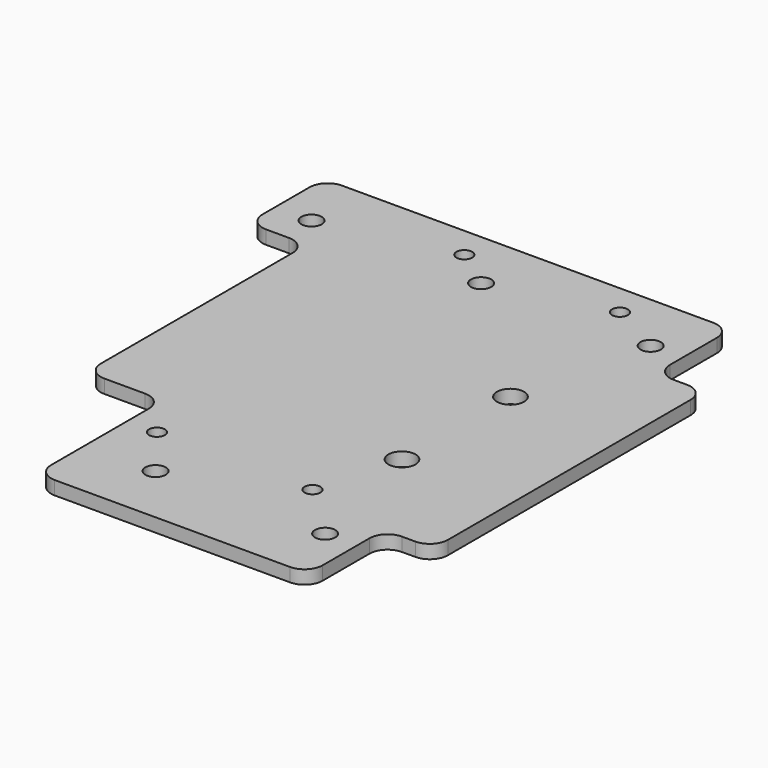
from build123d import *

# Parameters (mm, degrees)
F1_R     = 2.25
F1_R_2   = 1.75
F1_R_3   = 3
F2_DEPTH = 3
F3_W     = 17
F3_H     = 35
F4_DEPTH = 3.001
F5_R     = 4


with BuildPart() as f2:
    # F1 (on Top) → F2 (new body)
    with BuildSketch(Plane.XY):
        Polygon((44.55, 58.5), (-32.5, 58.5), (-45.55, 58.5), (-45.55, 37.5), (-32.5, 37.5), (-32.5, 0), (-32.5, -58.5), (44.55, -58.5), (44.55, -37.55), (55.5, -37.55), (55.5, 37.55), (44.55, 37.55), align=None)
        with Locations((0, -45)):
            Circle(F1_R, mode=Mode.SUBTRACT)
        with Locations((-8.9, -33.5)):
            Circle(F1_R_2, mode=Mode.SUBTRACT)
        with Locations((25.5, -33.5)):
            Circle(F1_R_2, mode=Mode.SUBTRACT)
        with Locations((37.5, -45)):
            Circle(F1_R, mode=Mode.SUBTRACT)
        with Locations((30.5, -15)):
            Circle(F1_R_3, mode=Mode.SUBTRACT)
        with Locations((-37.5, 45)):
            Circle(F1_R, mode=Mode.SUBTRACT)
        with Locations((-8.9, 51.5)):
            Circle(F1_R_2, mode=Mode.SUBTRACT)
        with Locations((0, 45)):
            Circle(F1_R, mode=Mode.SUBTRACT)
        with Locations((30.5, 15)):
            Circle(F1_R_3, mode=Mode.SUBTRACT)
        with Locations((25.5, 51.5)):
            Circle(F1_R_2, mode=Mode.SUBTRACT)
        with Locations((37.5, 45)):
            Circle(F1_R, mode=Mode.SUBTRACT)
    extrude(amount=F2_DEPTH)

    # F3 (on Top) → F4 (cut, through all)
    with BuildSketch(Plane.XY):
        with Locations((-24, -41)):
            Rectangle(F3_W, F3_H)
    extrude(amount=F4_DEPTH, mode=Mode.SUBTRACT)

    # F5
    f5_edges = [f2.edges().sort_by_distance(p)[0] for p in [
        (-45.55, 37.5, 1.5),
        (-45.55, 58.5, 1.5),
        (-32.5, 37.5, 1.5),
        (-32.5, -23.5, 1.5),
        (-15.5, -58.5, 1.5),
        (-15.5, -23.5, 1.5),
        (44.55, -58.5, 1.5),
        (44.55, -37.55, 1.5),
        (55.5, -37.55, 1.5),
        (55.5, 37.55, 1.5),
        (44.55, 37.55, 1.5),
        (44.55, 58.5, 1.5),
    ]]
    fillet(f5_edges, radius=F5_R)


solid = f2.part
